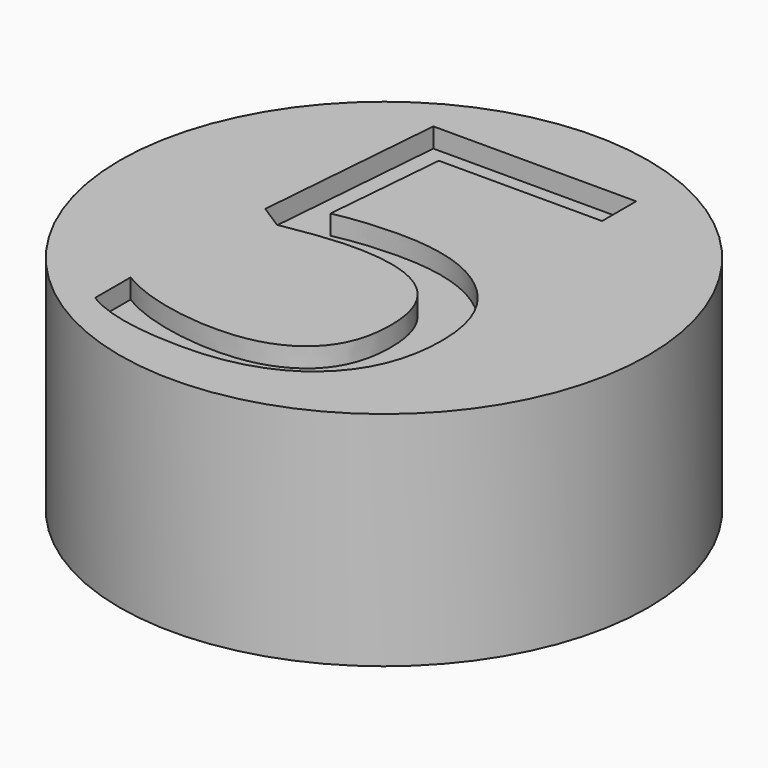
from build123d import *

# Parameters (mm, degrees)
F0_R         = 13.5
F1_DEPTH     = 11.35
F2_TEXT_SIZE = 29.2109534066
F3_DEPTH     = 1


# Not quite as in the source:
# - Text() gives the source's letters only with a copy of the font that has no kerning and outlines rounded to 1/6400 em; it was checked with that copy


with BuildPart() as f1:
    # F0 (on Top) → F1 (new body)
    with BuildSketch(Plane.XY):
        Circle(F0_R)
    extrude(amount=F1_DEPTH)

    # F2 (on face) → F3 (cut)
    with BuildSketch(Plane.XY.offset(11.35)):
        with Locations((-8.7447563537, -10.7469831321)):
            Text('5', F2_TEXT_SIZE, font='Open Sans', text_align=(TextAlign.LEFT, TextAlign.BOTTOM))
    extrude(amount=-F3_DEPTH, mode=Mode.SUBTRACT)


solid = f1.part
